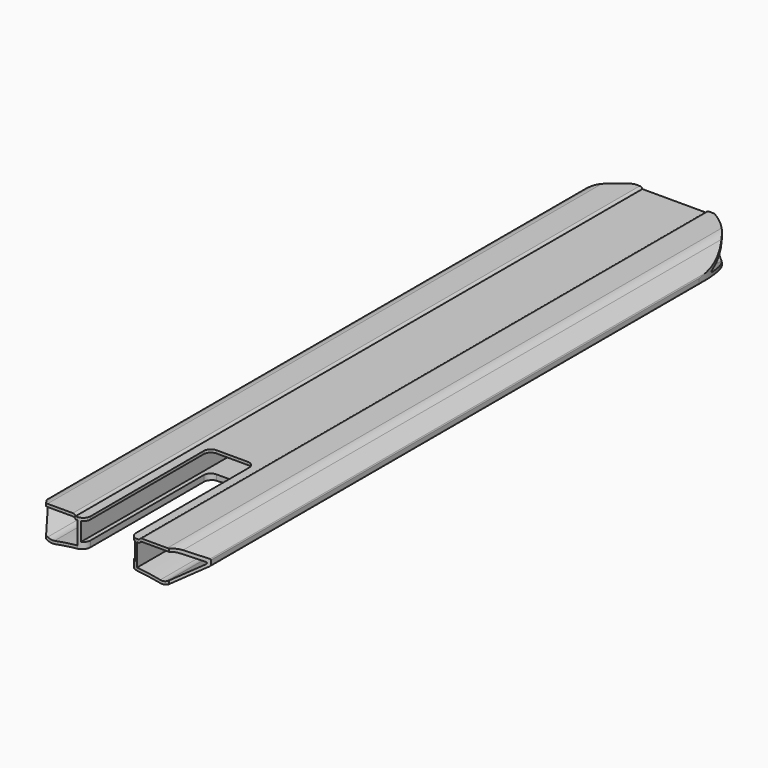
from build123d import *

# Parameters (mm, degrees)
F1_DEPTH       = 250
F2_W           = 38
F2_H           = 13
F3_DEPTH       = 250
F4_T1_DEPTH    = 509.3674969976
F5_R           = 9
F6_R           = 1
F8_DEPTH       = 500.001
F10_DEPTH      = 10.482205926
F10_DEPTH_BACK = 13.0380992553
F12_DEPTH      = 13.0380993553
F12_DEPTH_BACK = 10.4822060387
F13_F1_R       = 4.9999
F13_F2_R       = 5
F13_F3_R       = 5
F13_F4_R       = 4.9999
F13_F5_R       = 5
F13_F6_R       = 5


# Not quite as in the source:
# - a fillet or chamfer that OpenCascade refuses, or shapes differently, is made with other operations: its cross-section is extruded or revolved along the edge and cut away or added
# - a fillet or chamfer is up to 0.001 mm smaller than in the source, because OpenCascade refuses the exact size


with BuildPart() as f1:
    # F0 (on Front) → F1 (new body, symmetric)
    with BuildSketch(Plane.XZ):
        with BuildLine():
            Line((22.5, 11.7370992553), (0, 11.7370992553))
            Line((0, 11.7370992553), (-22.5, 11.7370992553))
            Line((-22.5, 11.7370992553), (-22.5, 13.0370992553))
            Line((-22.5, 13.0370992553), (-45.5824640741, 13.0370992553))
            Line((-45.5824640741, 13.0370992553), (-57.5, 3.0370992553))
            Line((-57.5, 3.0370992553), (-57.5, -0.9629007447))
            Line((-57.5, -0.9629007447), (-40.1794919243, -10.9629007447))
            ThreePointArc((-40.1794919243, -10.9629007447), (0, -6.8853558863), (40.1794919243, -10.9629007447))
            Line((40.1794919243, -10.9629007447), (57.5, -0.9629007447))
            Line((57.5, -0.9629007447), (57.5, 3.0370992553))
            Line((57.5, 3.0370992553), (45.5824640741, 13.0370992553))
            Line((45.5824640741, 13.0370992553), (22.5, 13.0370992553))
            Line((22.5, 13.0370992553), (22.5, 11.7370992553))
        make_face()
    extrude(amount=F1_DEPTH, both=True)

    # F2 (on Front) → F3 (cut, symmetric)
    with BuildSketch(Plane.XZ):
        with Locations((0, 3.2370992553)):
            Rectangle(F2_W, F2_H)
    extrude(amount=F3_DEPTH, both=True, mode=Mode.SUBTRACT)

    # F4: fillet of radius 2 on 2 edges, made by hand

    # F4_s2 → F4_t1 (cut)
    with BuildSketch(Plane.XZ.offset(-254.6837484988)):
        with BuildLine():
            ThreePointArc((-22.5, 11.7370992553), (-23.2333239744, 12.6802669278), (-24.3734993995, 13.0370992553))
            Line((-24.3734993995, 13.0370992553), (-22.5, 13.0370992553))
            Line((-22.5, 13.0370992553), (-22.5, 11.7370992553))
        make_face()
        with BuildLine():
            ThreePointArc((24.3734993995, 13.0370992553), (23.2333239744, 12.6802669278), (22.5, 11.7370992553))
            Line((22.5, 11.7370992553), (22.5, 13.0370992553))
            Line((22.5, 13.0370992553), (24.3734993995, 13.0370992553))
        make_face()
    extrude(amount=F4_T1_DEPTH, mode=Mode.SUBTRACT)

    # F5
    f5_edges = [f1.edges().sort_by_distance(p)[0] for p in [
        (-45.582464, 0, 13.037099),
        (45.582464, 0, 13.037099),
        (-40.179492, 0, -10.962901),
        (40.179492, 0, -10.962901),
    ]]
    fillet(f5_edges, radius=F5_R)

    # F6
    f6_edges = [f1.edges().sort_by_distance(p)[0] for p in [
        (57.5, 0, 3.037099),
        (57.5, 0, -0.962901),
        (-57.5, 0, 3.037099),
        (-57.5, 0, -0.962901),
    ]]
    fillet(f6_edges, radius=F6_R)

    # F7 (on face) → F8 (cut, through all)
    with BuildSketch(Plane.XZ.offset(250)):
        with BuildLine():
            ThreePointArc((-42.1022690923, -7.5433837525), (-39.7790673433, -8.3815788055), (-37.3093701274, -8.3607707572))
            ThreePointArc((-37.3093701274, -8.3607707572), (-29.1789785809, -7.0039230093), (-21, -5.9799054874))
            Line((-21, -5.9799054874), (-21, 9.7370992553))
            Line((-21, 9.7370992553), (-22.5, 9.7370992553))
            ThreePointArc((-22.5, 9.7370992553), (-23.2333239744, 10.6802669278), (-24.3734993995, 11.0370992553))
            Line((-24.3734993995, 11.0370992553), (-42.3067319657, 11.0370992553))
            ThreePointArc((-42.3067319657, 11.0370992553), (-44.7008729689, 10.6149476008), (-46.8062452335, 9.3994103571))
            Line((-46.8062452335, 9.3994103571), (-55.7563117574, 1.8894128378))
            ThreePointArc((-55.7563117574, 1.8894128378), (-56.1097188459, 1.036212652), (-55.6135241478, 0.2573429909))
            Line((-55.6135241478, 0.2573429909), (-42.1022690923, -7.5433837525))
        make_face()
        with BuildLine():
            Line((55.7563117574, 1.8894128378), (46.8062452335, 9.3994103571))
            ThreePointArc((46.8062452335, 9.3994103571), (44.7008729689, 10.6149476008), (42.3067319657, 11.0370992553))
            Line((42.3067319657, 11.0370992553), (24.3734993995, 11.0370992553))
            ThreePointArc((24.3734993995, 11.0370992553), (23.2333239744, 10.6802669278), (22.5, 9.7370992553))
            Line((22.5, 9.7370992553), (21, 9.7370992553))
            Line((21, 9.7370992553), (21, -5.9799054874))
            ThreePointArc((21, -5.9799054874), (29.1789785809, -7.0039230093), (37.3093701274, -8.3607707572))
            ThreePointArc((37.3093701274, -8.3607707572), (39.7790673433, -8.3815788055), (42.1022690923, -7.5433837525))
            Line((42.1022690923, -7.5433837525), (55.6135241478, 0.2573429909))
            ThreePointArc((55.6135241478, 0.2573429909), (56.1097188459, 1.036212652), (55.7563117574, 1.8894128378))
        make_face()
    extrude(amount=-F8_DEPTH, mode=Mode.SUBTRACT)

    # F9 (on Top) → F10 (cut, two sides)
    with BuildSketch(Plane.XY) as f10_sk:
        with BuildLine():
            ThreePointArc((-57.5, 200), (0, 257.5), (57.5, 200))
            Line((57.5, 200), (57.5, 280))
            Line((57.5, 280), (-57.5, 280))
            Line((-57.5, 280), (-57.5, 200))
        make_face()
    extrude(amount=-F10_DEPTH, mode=Mode.SUBTRACT)
    extrude(f10_sk.sketch, amount=F10_DEPTH_BACK, mode=Mode.SUBTRACT)

    # F11 (on Top) → F12 (cut, two sides)
    with BuildSketch(Plane.XY) as f12_sk:
        Polygon((16, -140), (-16, -140), (-16, -250), (-43.2975540478, -250), (-68, -216), (-68, -346), (68, -346), (68, -216), (43.2975540478, -250), (16, -250), align=None)
    extrude(amount=F12_DEPTH, mode=Mode.SUBTRACT)
    extrude(f12_sk.sketch, amount=-F12_DEPTH_BACK, mode=Mode.SUBTRACT)

    # F13: fillet of radius 5 on 8 edges, made by hand

    # F13_f1 (radius 5 in the source; OpenCascade refuses exactly that, so slightly less here)
    f13_f1_edges = [f1.edges().sort_by_distance(p)[0] for p in [
        (16, -250, -5.3946419605),
    ]]
    fillet(f13_f1_edges, radius=F13_F1_R)

    # F13_f2
    f13_f2_edges = [f1.edges().sort_by_distance(p)[0] for p in [
        (16, -140, -5.3946419605),
    ]]
    fillet(f13_f2_edges, radius=F13_F2_R)

    # F13_f3
    f13_f3_edges = [f1.edges().sort_by_distance(p)[0] for p in [
        (16, -140, 10.7370992553),
    ]]
    fillet(f13_f3_edges, radius=F13_F3_R)

    # F13_f4 (radius 5 in the source; OpenCascade refuses exactly that, so slightly less here)
    f13_f4_edges = [f1.edges().sort_by_distance(p)[0] for p in [
        (-16, -250, 10.7370992553),
    ]]
    fillet(f13_f4_edges, radius=F13_F4_R)

    # F13_f5
    f13_f5_edges = [f1.edges().sort_by_distance(p)[0] for p in [
        (-16, -140, -5.3946419605),
    ]]
    fillet(f13_f5_edges, radius=F13_F5_R)

    # F13_f6
    f13_f6_edges = [f1.edges().sort_by_distance(p)[0] for p in [
        (-16, -140, 10.7370992553),
    ]]
    fillet(f13_f6_edges, radius=F13_F6_R)


solid = f1.part
